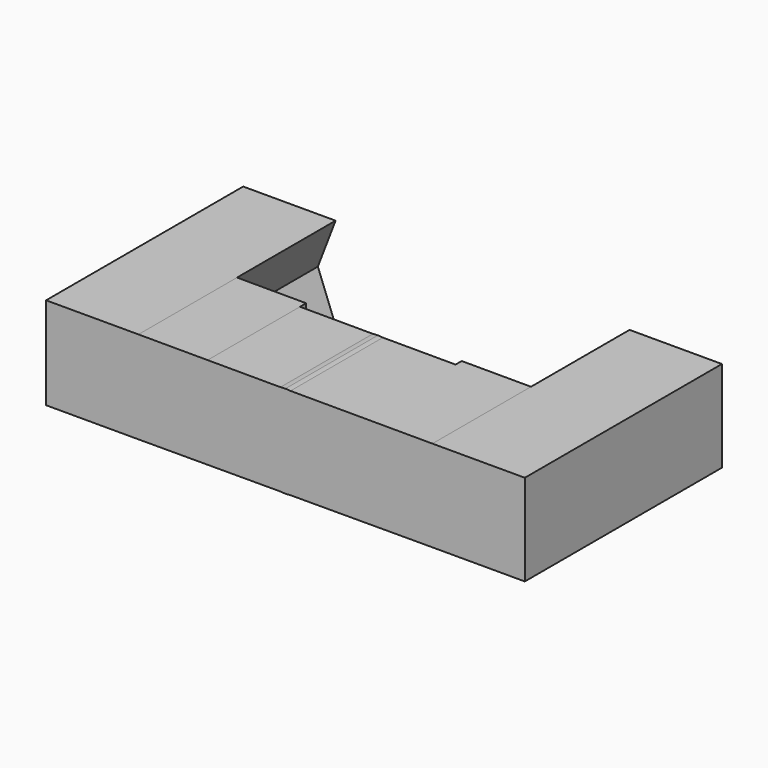
from build123d import *

# Parameters (mm, degrees)
F1_DEPTH = 8
F2_DEPTH = 4
F3_DEPTH = 4.25


# Not quite as in the source:
# - a feature of the source that left no trace in its solid (it failed there, or was rolled back) is left out


with BuildPart() as f1:
    # F0 (on Front) → F1 (new body)
    with BuildSketch(Plane.XZ):
        with BuildLine():
            Line((2.5197209473, -1.4865167008), (2.5252201747, 1.4865065289))
            Line((2.5252201747, 1.4865065289), (0.1652307775, 1.4908718222))
            ThreePointArc((0.1652307775, 1.4908718222), (1.1175522731, 1.0005383135), (1.5, 0))
            ThreePointArc((1.5, 0), (1.1175522731, -1.0005383135), (0.1652307775, -1.4908718222))
            Line((0.1652307775, -1.4908718222), (2.5197209473, -1.4865167008))
        make_face()
        Polygon((-5.3444080986, 0), (-4.7696960071, 1.5), (-7.7696960071, 1.5), (-7.7696960071, -1.5), (-4.7696960071, -1.5), align=None)
        Polygon((7.7752124765, 1.4823446982), (4.7752124765, 1.4823446982), (5.3444080986, 0), (4.7752124765, -1.4823446982), (7.7752124765, -1.4823446982), align=None)
        with BuildLine():
            ThreePointArc((-4.7696960071, -1.5), (-5, 0), (-4.7696960071, 1.5))
            Line((-4.7696960071, 1.5), (-5.3444080986, 0))
            Line((-5.3444080986, 0), (-4.7696960071, -1.5))
        make_face()
        with BuildLine():
            Line((5.3444080986, 0), (4.7752124765, 1.4823446982))
            ThreePointArc((4.7752124765, 1.4823446982), (4.94348371, 0.7496457888), (5, 0))
            ThreePointArc((5, 0), (4.94348371, -0.7496457888), (4.7752124765, -1.4823446982))
            Line((4.7752124765, -1.4823446982), (5.3444080986, 0))
        make_face()
        with BuildLine():
            Line((-2.5252374544, 1.4958484051), (-4.7696960071, 1.5))
            ThreePointArc((-4.7696960071, 1.5), (-5, 0), (-4.7696960071, -1.5))
            Line((-4.7696960071, -1.5), (-2.5197037053, -1.4958381693))
            Line((-2.5197037053, -1.4958381693), (-2.5252374544, 1.4958484051))
        make_face()
        with BuildLine():
            ThreePointArc((5, 0), (4.94348371, 0.7496457888), (4.7752124765, 1.4823446982))
            Line((4.7752124765, 1.4823446982), (2.5252201747, 1.4865065289))
            Line((2.5252201747, 1.4865065289), (2.5197209473, -1.4865167008))
            Line((2.5197209473, -1.4865167008), (4.7752124765, -1.4823446982))
            ThreePointArc((4.7752124765, -1.4823446982), (4.94348371, -0.7496457888), (5, 0))
        make_face()
        with BuildLine():
            Line((0, 1.491177451), (-0.1597143081, 1.491472876))
            ThreePointArc((-0.1597143081, 1.491472876), (-1.5, 0), (-0.1597143081, -1.491472876))
            Line((-0.1597143081, -1.491472876), (0, -1.491177451))
            Line((0, -1.491177451), (0, 1.491177451))
        make_face()
        with BuildLine():
            Line((-0.1597143081, 1.491472876), (-2.5252374544, 1.4958484051))
            Line((-2.5252374544, 1.4958484051), (-2.5197037053, -1.4958381693))
            Line((-2.5197037053, -1.4958381693), (-0.1597143081, -1.491472876))
            ThreePointArc((-0.1597143081, -1.491472876), (-1.5, 0), (-0.1597143081, 1.491472876))
        make_face()
        with BuildLine():
            ThreePointArc((1.5, 0), (1.1175522731, 1.0005383135), (0.1652307775, 1.4908718222))
            Line((0.1652307775, 1.4908718222), (0, 1.491177451))
            Line((0, 1.491177451), (0, -1.491177451))
            Line((0, -1.491177451), (0.1652307775, -1.4908718222))
            ThreePointArc((0.1652307775, -1.4908718222), (1.1175522731, -1.0005383135), (1.5, 0))
        make_face()
        with BuildLine():
            Line((0, 1.491177451), (0.1652307775, 1.4908718222))
            ThreePointArc((0.1652307775, 1.4908718222), (0.0827413643, 1.497716217), (0, 1.5))
            Line((0, 1.5), (0, 1.491177451))
        make_face()
        with BuildLine():
            ThreePointArc((0, 1.5), (-0.0799708885, 1.497866702), (-0.1597143081, 1.491472876))
            Line((-0.1597143081, 1.491472876), (0, 1.491177451))
            Line((0, 1.491177451), (0, 1.5))
        make_face()
        with BuildLine():
            Line((0, -1.491177451), (-0.1597143081, -1.491472876))
            ThreePointArc((-0.1597143081, -1.491472876), (-0.0799708885, -1.497866702), (0, -1.5))
            Line((0, -1.5), (0, -1.491177451))
        make_face()
        with BuildLine():
            ThreePointArc((0, -1.5), (0.0827413643, -1.497716217), (0.1652307775, -1.4908718222))
            Line((0.1652307775, -1.4908718222), (0, -1.491177451))
            Line((0, -1.491177451), (0, -1.5))
        make_face()
    extrude(amount=F1_DEPTH)

    # F0 (on Front) → F2 (cut)
    with BuildSketch(Plane.XZ):
        with BuildLine():
            Line((5.3444080986, 0), (4.7752124765, 1.4823446982))
            ThreePointArc((4.7752124765, 1.4823446982), (4.94348371, 0.7496457888), (5, 0))
            ThreePointArc((5, 0), (4.94348371, -0.7496457888), (4.7752124765, -1.4823446982))
            Line((4.7752124765, -1.4823446982), (5.3444080986, 0))
        make_face()
        with BuildLine():
            ThreePointArc((5, 0), (4.94348371, 0.7496457888), (4.7752124765, 1.4823446982))
            Line((4.7752124765, 1.4823446982), (2.5252201747, 1.4865065289))
            Line((2.5252201747, 1.4865065289), (2.5197209473, -1.4865167008))
            Line((2.5197209473, -1.4865167008), (4.7752124765, -1.4823446982))
            ThreePointArc((4.7752124765, -1.4823446982), (4.94348371, -0.7496457888), (5, 0))
        make_face()
        with BuildLine():
            Line((2.5197209473, -1.4865167008), (2.5252201747, 1.4865065289))
            Line((2.5252201747, 1.4865065289), (0.1652307775, 1.4908718222))
            ThreePointArc((0.1652307775, 1.4908718222), (1.1175522731, 1.0005383135), (1.5, 0))
            ThreePointArc((1.5, 0), (1.1175522731, -1.0005383135), (0.1652307775, -1.4908718222))
            Line((0.1652307775, -1.4908718222), (2.5197209473, -1.4865167008))
        make_face()
        with BuildLine():
            ThreePointArc((1.5, 0), (1.1175522731, 1.0005383135), (0.1652307775, 1.4908718222))
            Line((0.1652307775, 1.4908718222), (0, 1.491177451))
            Line((0, 1.491177451), (0, -1.491177451))
            Line((0, -1.491177451), (0.1652307775, -1.4908718222))
            ThreePointArc((0.1652307775, -1.4908718222), (1.1175522731, -1.0005383135), (1.5, 0))
        make_face()
        with BuildLine():
            Line((0, 1.491177451), (-0.1597143081, 1.491472876))
            ThreePointArc((-0.1597143081, 1.491472876), (-1.5, 0), (-0.1597143081, -1.491472876))
            Line((-0.1597143081, -1.491472876), (0, -1.491177451))
            Line((0, -1.491177451), (0, 1.491177451))
        make_face()
        with BuildLine():
            Line((-0.1597143081, 1.491472876), (-2.5252374544, 1.4958484051))
            Line((-2.5252374544, 1.4958484051), (-2.5197037053, -1.4958381693))
            Line((-2.5197037053, -1.4958381693), (-0.1597143081, -1.491472876))
            ThreePointArc((-0.1597143081, -1.491472876), (-1.5, 0), (-0.1597143081, 1.491472876))
        make_face()
        with BuildLine():
            Line((-2.5252374544, 1.4958484051), (-4.7696960071, 1.5))
            ThreePointArc((-4.7696960071, 1.5), (-5, 0), (-4.7696960071, -1.5))
            Line((-4.7696960071, -1.5), (-2.5197037053, -1.4958381693))
            Line((-2.5197037053, -1.4958381693), (-2.5252374544, 1.4958484051))
        make_face()
        with BuildLine():
            ThreePointArc((-4.7696960071, -1.5), (-5, 0), (-4.7696960071, 1.5))
            Line((-4.7696960071, 1.5), (-5.3444080986, 0))
            Line((-5.3444080986, 0), (-4.7696960071, -1.5))
        make_face()
    extrude(amount=F2_DEPTH, mode=Mode.SUBTRACT)

    # F0 (on Front) → F3 (cut)
    with BuildSketch(Plane.XZ):
        with BuildLine():
            Line((2.5197209473, -1.4865167008), (2.5252201747, 1.4865065289))
            Line((2.5252201747, 1.4865065289), (0.1652307775, 1.4908718222))
            ThreePointArc((0.1652307775, 1.4908718222), (1.1175522731, 1.0005383135), (1.5, 0))
            ThreePointArc((1.5, 0), (1.1175522731, -1.0005383135), (0.1652307775, -1.4908718222))
            Line((0.1652307775, -1.4908718222), (2.5197209473, -1.4865167008))
        make_face()
        with BuildLine():
            ThreePointArc((1.5, 0), (1.1175522731, 1.0005383135), (0.1652307775, 1.4908718222))
            Line((0.1652307775, 1.4908718222), (0, 1.491177451))
            Line((0, 1.491177451), (0, -1.491177451))
            Line((0, -1.491177451), (0.1652307775, -1.4908718222))
            ThreePointArc((0.1652307775, -1.4908718222), (1.1175522731, -1.0005383135), (1.5, 0))
        make_face()
        with BuildLine():
            Line((-0.1597143081, 1.491472876), (-2.5252374544, 1.4958484051))
            Line((-2.5252374544, 1.4958484051), (-2.5197037053, -1.4958381693))
            Line((-2.5197037053, -1.4958381693), (-0.1597143081, -1.491472876))
            ThreePointArc((-0.1597143081, -1.491472876), (-1.5, 0), (-0.1597143081, 1.491472876))
        make_face()
        with BuildLine():
            Line((0, 1.491177451), (-0.1597143081, 1.491472876))
            ThreePointArc((-0.1597143081, 1.491472876), (-1.5, 0), (-0.1597143081, -1.491472876))
            Line((-0.1597143081, -1.491472876), (0, -1.491177451))
            Line((0, -1.491177451), (0, 1.491177451))
        make_face()
        with BuildLine():
            ThreePointArc((0, 1.5), (-0.0799708885, 1.497866702), (-0.1597143081, 1.491472876))
            Line((-0.1597143081, 1.491472876), (0, 1.491177451))
            Line((0, 1.491177451), (0, 1.5))
        make_face()
        with BuildLine():
            Line((0, 1.491177451), (0.1652307775, 1.4908718222))
            ThreePointArc((0.1652307775, 1.4908718222), (0.0827413643, 1.497716217), (0, 1.5))
            Line((0, 1.5), (0, 1.491177451))
        make_face()
        with BuildLine():
            ThreePointArc((0, -1.5), (0.0827413643, -1.497716217), (0.1652307775, -1.4908718222))
            Line((0.1652307775, -1.4908718222), (0, -1.491177451))
            Line((0, -1.491177451), (0, -1.5))
        make_face()
        with BuildLine():
            Line((0, -1.491177451), (-0.1597143081, -1.491472876))
            ThreePointArc((-0.1597143081, -1.491472876), (-0.0799708885, -1.497866702), (0, -1.5))
            Line((0, -1.5), (0, -1.491177451))
        make_face()
    extrude(amount=F3_DEPTH, mode=Mode.SUBTRACT)


solid = f1.part
